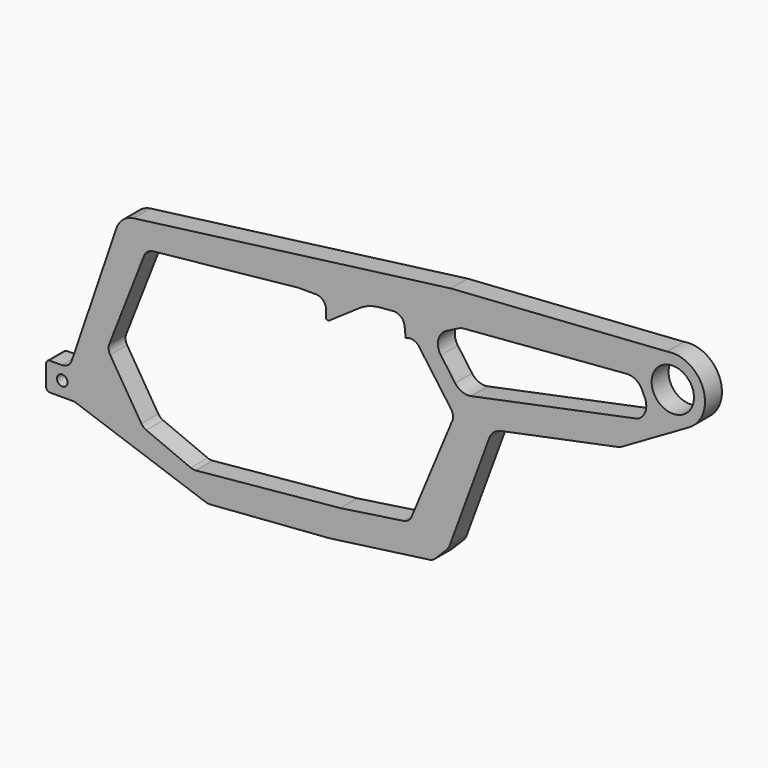
from build123d import *

# Parameters (mm, degrees)
F1_R     = 1
F1_R_2   = 4
F2_DEPTH = 4


# Not quite as in the source:
# - a feature names something its author has since deleted; it is built from what else it names


with BuildPart() as f2:
    # F1 (on Front) → F2 (new body)
    with BuildSketch(Plane.XZ):
        with BuildLine():
            ThreePointArc((54.0977004839, -4.1335701552), (56.766858502, 3.238282099), (49.9672364551, 7.1413258089))
            Line((49.9672364551, 7.1413258089), (9.0970295176, 4.3491148777))
            Line((9.0970295176, 4.3491148777), (-50.8374237274, -3.466212469))
            ThreePointArc((-50.8374237274, -3.466212469), (-52.8544943464, -4.3378942821), (-54.1067810637, -6.1434914253))
            Line((-54.1067810637, -6.1434914253), (-62.5583549212, -30.968136056))
            ThreePointArc((-62.5583549212, -30.968136056), (-63.2874110026, -31.9497789492), (-64.4516400514, -32.3235653341))
            Line((-64.4516400514, -32.3235653341), (-66.6727852076, -32.3235653341))
            ThreePointArc((-66.6727852076, -32.3235653341), (-67.1968351707, -32.5406339362), (-67.4139037728, -33.0646838993))
            Line((-67.4139037728, -33.0646838993), (-67.4139037728, -36.8838813156))
            ThreePointArc((-67.4139037728, -36.8838813156), (-67.1968351707, -37.4079312787), (-66.6727852076, -37.6249998808))
            Line((-66.6727852076, -37.6249998808), (-62.3935461021, -37.6249998808))
            ThreePointArc((-62.3935461021, -37.6249998808), (-62.0598715448, -37.6530309942), (-61.7355502568, -37.736338591))
            Line((-61.7355502568, -37.736338591), (-37.2162681051, -46.2786780104))
            ThreePointArc((-37.2162681051, -46.2786780104), (-36.8173856222, -46.3731607561), (-36.4076181612, -46.3843344843))
            Line((-36.4076181612, -46.3843344843), (-13.7597462162, -44.6734763682))
            Line((-13.7597462162, -44.6734763682), (5.0197247755, -42.1101055891))
            ThreePointArc((5.0197247755, -42.1101055891), (5.6431122997, -41.9176107253), (6.1713765615, -41.5347228206))
            Line((6.1713765615, -41.5347228206), (8.2269536442, -39.4559054448))
            ThreePointArc((8.2269536442, -39.4559054448), (8.625280402, -38.9562994549), (8.9087680688, -38.3836694749))
            Line((8.9087680688, -38.3836694749), (16.3488967626, -18.1892685938))
            ThreePointArc((16.3488967626, -18.1892685938), (17.208766797, -16.9510123668), (18.5623472371, -16.2873294968))
            Line((18.5623472371, -16.2873294968), (40.5820753294, -11.7802791422))
            ThreePointArc((40.5820753294, -11.7802791422), (41.0467937044, -11.6453208131), (41.4837674916, -11.4374005686))
            Line((41.4837674916, -11.4374005686), (54.0977004839, -4.1335701552))
        make_face()
        with Locations((-64.3514022231, -34.8506011069)):
            Circle(F1_R, mode=Mode.SUBTRACT)
        with BuildLine():
            ThreePointArc((-16.7472230261, -4.91411715), (-15.1379574632, -5.4133219884), (-14.4811960302, -6.9649680637))
            Line((-14.4811960302, -6.9649680637), (-14.5219445245, -8.1491333606))
            ThreePointArc((-14.5219445245, -8.1491333606), (-14.32171034, -8.5009617779), (-13.9174035461, -8.4806398607))
            Line((-13.9174035461, -8.4806398607), (-8.2003281839, -4.5523469385))
            ThreePointArc((-8.2003281839, -4.5523469385), (-6.3639342341, -3.6131535453), (-4.348447762, -3.1747002983))
            Line((-4.348447762, -3.1747002983), (-1.8018096929, -2.9578907207))
            ThreePointArc((-1.8018096929, -2.9578907207), (-0.3607692656, -3.4067953543), (0.3561826933, -4.7349868962))
            Line((0.3561826933, -4.7349868962), (0.5668963829, -6.67740348))
            Line((0.5668963829, -6.67740348), (0.672921323, -6.6315499412))
            ThreePointArc((0.672921323, -6.6315499412), (1.9999899765, -6.5396114649), (3.091186979, -7.3004353579))
            Line((3.091186979, -7.3004353579), (9.1316822834, -15.7097849605))
            ThreePointArc((9.1316822834, -15.7097849605), (9.4794348377, -16.5438272503), (9.4245987558, -17.4457980836))
            ThreePointArc((9.4245987558, -17.4457980836), (9.3536544385, -17.6453573177), (9.2620047676, -17.8362953231))
            Line((9.2620047676, -17.8362953231), (4.5568440785, -29.1365425288))
            Line((4.5568440785, -29.1365425288), (3.6719114619, -31.2618593858))
            ThreePointArc((3.6719114619, -31.2618593858), (3.5914700409, -31.4944450482), (3.483071784, -31.715390133))
            Line((3.483071784, -31.715390133), (1.6890171815, -36.0241187498))
            ThreePointArc((1.6890171815, -36.0241187498), (1.0710114326, -36.8336930562), (0.1344541234, -37.2339455637))
            Line((0.1344541234, -37.2339455637), (-11.7459257638, -38.985923444))
            Line((-11.7459257638, -38.985923444), (-39.1007720975, -41.6174277811))
            ThreePointArc((-39.1007720975, -41.6174277811), (-39.5919940555, -41.6040344694), (-40.0651227377, -41.4712653355))
            Line((-40.0651227377, -41.4712653355), (-48.4746967713, -37.9479731273))
            ThreePointArc((-48.4746967713, -37.9479731273), (-48.9998078369, -37.6249470931), (-49.401585452, -37.1573337934))
            Line((-49.401585452, -37.1573337934), (-55.2931292161, -27.6564465473))
            ThreePointArc((-55.2931292161, -27.6564465473), (-55.5850730561, -26.7847906202), (-55.4562690933, -25.874612176))
            Line((-55.4562690933, -25.874612176), (-48.8776308187, -9.0366472667))
            ThreePointArc((-48.8776308187, -9.0366472667), (-48.2268856759, -8.1736364118), (-47.2221234757, -7.7752523038))
            Line((-47.2221234757, -7.7752523038), (-19.7747927159, -4.91411715))
            Line((-19.7747927159, -4.91411715), (-16.7472230261, -4.91411715))
        make_face(mode=Mode.SUBTRACT)
        with BuildLine():
            ThreePointArc((7.2113401452, -7.3855209262), (6.7341998146, -4.9209260348), (8.2972601063, -2.9565601324))
            Line((8.2972601063, -2.9565601324), (10.5244084197, -1.8336281786))
            ThreePointArc((10.5244084197, -1.8336281786), (11.0639592867, -1.6241164689), (11.6337015289, -1.5221161154))
            Line((11.6337015289, -1.5221161154), (42.2805400914, 0.9513819838))
            ThreePointArc((42.2805400914, 0.9513819838), (44.1319918409, 0.4924203394), (45.3325095049, -0.989901053))
            ThreePointArc((45.3325095049, -0.989901053), (45.4924194241, -1.3771741585), (45.6785557512, -1.752547184))
            ThreePointArc((45.6785557512, -1.752547184), (45.9010642846, -4.0736832448), (44.3940516522, -5.8530358197))
            Line((44.3940516522, -5.8530358197), (12.9439963939, -12.3211824174))
            ThreePointArc((12.9439963939, -12.3211824174), (11.2477431433, -12.1769167526), (9.9030954921, -11.132881137))
            Line((9.9030954921, -11.132881137), (7.2113401452, -7.3855209262))
        make_face(mode=Mode.SUBTRACT)
        with Locations((51.0432839383, 1.1414983302)):
            Circle(F1_R_2, mode=Mode.SUBTRACT)
    extrude(amount=F2_DEPTH)


solid = f2.part
